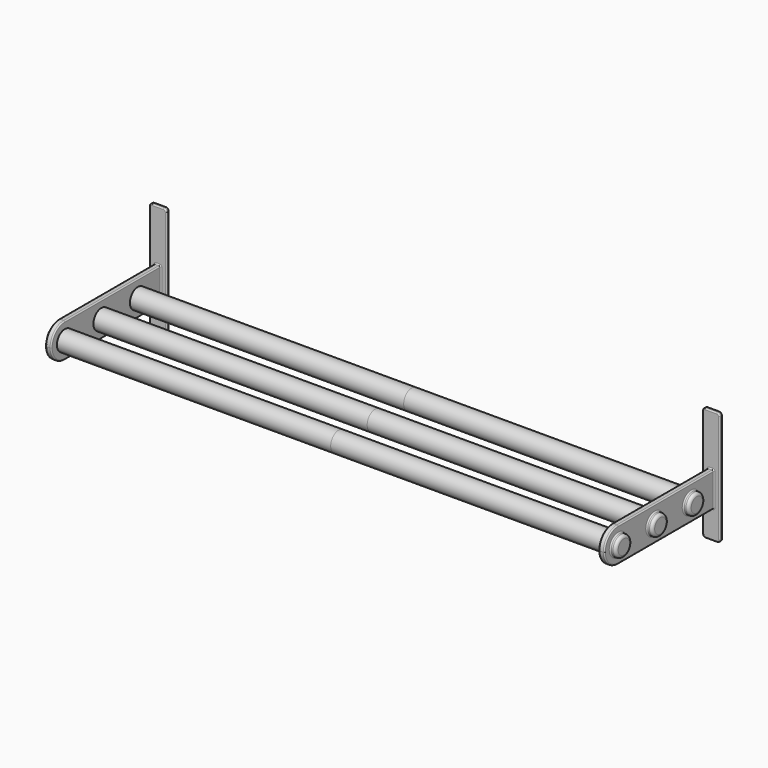
from build123d import *

# Parameters (mm, degrees)
F0_W     = 5
F0_H     = 200
F1_DEPTH = 30
F2_W     = 10
F2_H     = 60
F3_DEPTH = 240
F4_R     = 29.99999
F5_R     = 17.5
F6_DEPTH = 10
F7_R     = 17.5
F8_DEPTH = 490
F9_R     = 5
F10_R    = 2


# Not quite as in the source:
# - a fillet or chamfer is up to 0.001 mm smaller than in the source, because OpenCascade refuses the exact size


with BuildPart() as f1:
    # F0 (on Right) → F1 (new body)
    with BuildSketch(Plane.YZ):
        with Locations((2.5, 100)):
            Rectangle(F0_W, F0_H)
    extrude(amount=F1_DEPTH)

    # F2 (on face) → F3 (join)
    with BuildSketch(Plane.XZ):
        with Locations((15, 80)):
            Rectangle(F2_W, F2_H)
    extrude(amount=F3_DEPTH)

    # F4 (radius 30 in the source; OpenCascade refuses exactly that, so slightly less here)
    f4_edges = [f1.edges().sort_by_distance(p)[0] for p in [
        (15, -240, 110),
        (15, -240, 50),
    ]]
    fillet(f4_edges, radius=F4_R)

    # F5 (on face) → F6 (join)
    with BuildSketch(Plane(origin=(10, 0, 0), x_dir=(0, -1, 0), z_dir=(-1, 0, 0))):
        with Locations((210, 80)):
            Circle(F5_R)
        with Locations((130, 80)):
            Circle(F5_R)
        with Locations((50, 80)):
            Circle(F5_R)
    extrude(amount=F6_DEPTH)

    # F7 (on face) → F8 (join)
    with BuildSketch(Plane(origin=(10, 0, 0), x_dir=(0, -1, 0), z_dir=(-1, 0, 0))):
        with Locations((50, 80)):
            Circle(F7_R)
        with Locations((130, 80)):
            Circle(F7_R)
        with Locations((210, 80)):
            Circle(F7_R)
    extrude(amount=-F8_DEPTH)

    # F9
    f9_edges = [f1.edges().sort_by_distance(p)[0] for p in [
        (0, -192.5, 80),
        (0, -112.5, 80),
        (0, -32.5, 80),
        (0, 2.5, 0),
        (30, 2.5, 0),
        (30, 2.5, 200),
        (0, 2.5, 200),
    ]]
    fillet(f9_edges, radius=F9_R)

    # F10
    f10_edges = [f1.edges().sort_by_distance(p)[0] for p in [
        (15, 0, 200),
        (1.464466, 0, 198.535534),
        (28.535534, 0, 198.535534),
        (0, 0, 100),
        (30, 0, 100),
        (1.464466, 0, 1.464466),
        (28.535534, 0, 1.464466),
        (15, 0, 0),
        (20, 0, 80),
        (15, 0, 50),
        (10, 0, 80),
        (15, 0, 110),
        (10, -105.000005, 110),
        (10, -231.213206, 101.213206),
        (10, -240, 80),
        (10, -105.000005, 50),
        (10, -231.213206, 58.786794),
        (10, -192.5, 80),
        (10, -112.5, 80),
        (10, -32.5, 80),
        (15, -210.00001, 50),
        (20, -105.000005, 50),
    ]]
    fillet(f10_edges, radius=F10_R)

    # F12: F1 across plane


with BuildPart() as f1_1:
    add(f1.part)
    add(f1.part.mirror(Plane.YZ.offset(500)))


solid = f1_1.part
